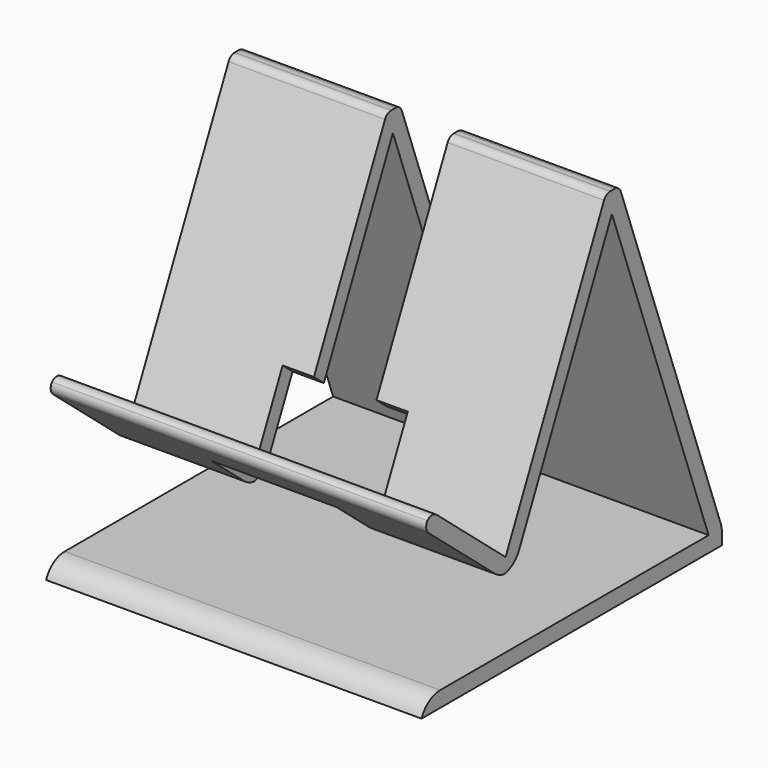
from build123d import *

# Parameters (mm, degrees)
F0_W        = 76.2
F0_H        = 76.2
F1_DEPTH    = 3.175
F3_DEPTH    = 76.2
F4_R        = 1.7145
F5_R        = 5.08
F6_T1_DEPTH = 84.7725
F7_T1_DEPTH = 92.3815846245
F7_T3_DEPTH = 85.4448439504
F8_T1_DEPTH = 99.7464301965
F9_W        = 12.7
F9_H        = 76.2
F10_REACH   = 149.9425757938
F11_W       = 25.4
F11_H       = 19.8840972021
F12_DEPTH   = 19.05
F14_DEPTH   = 0.5
F16_DEPTH   = 0.5


# Not quite as in the source:
# - a fillet or chamfer that OpenCascade refuses, or shapes differently, is made with other operations: its cross-section is extruded or revolved along the edge and cut away or added


with BuildPart() as f1:
    # F0 (on Top) → F1 (new body)
    with BuildSketch(Plane.XY):
        with Locations((-12.8260315396, -9.7117862726)):
            Rectangle(F0_W, F0_H)
    extrude(amount=F1_DEPTH)

    # F2 (on face) → F3 (join)
    with BuildSketch(Plane(origin=(-50.9260315396, 0, 0), x_dir=(0, -1, 0), z_dir=(-1, 0, 0))):
        Polygon((1.0524856216, 74.7795777039), (-0.4832286212, 70.560237499), (24.3855203494, 17.2290332271), (27.8887452421, 17.2290332271), (26.4995982243, 20.2080686204), align=None)
        Polygon((45.3054234366, 35.98802962), (26.4995982243, 20.2080686204), (27.8887452421, 17.2290332271), (47.3462740973, 33.5558385131), align=None)
        Polygon((-2.326278806, 74.7795777039), (-28.3882137274, 3.175), (-25.0094492998, 3.175), (-0.4832286212, 70.560237499), (1.0524856216, 74.7795777039), align=None)
    extrude(amount=-F3_DEPTH)

    # F4
    f4_edges = [f1.edges().sort_by_distance(p)[0] for p in [
        (-12.826032, -1.052486, 74.779578),
        (-12.826032, 2.326279, 74.779578),
    ]]
    fillet(f4_edges, radius=F4_R)

    # F5
    f5_edges = [f1.edges().sort_by_distance(p)[0] for p in [
        (-12.826032, 28.388214, 3.175),
    ]]
    fillet(f5_edges, radius=F5_R)

    # F6: fillet of radius 1.7145 on 2 edges, made by hand

    # F6_s2 → F6_t1 (cut)
    with BuildSketch(Plane.YZ.offset(-55.2122815396)):
        with BuildLine():
            ThreePointArc((-43.9920402389, 34.8859702632), (-45.2435281166, 35.2805628753), (-46.4074827934, 34.6746464223))
            Line((-46.4074827934, 34.6746464223), (-45.3054234366, 35.98802962))
            Line((-45.3054234366, 35.98802962), (-43.9920402389, 34.8859702632))
        make_face()
        with BuildLine():
            ThreePointArc((-46.2442147405, 34.8692217108), (-46.6388073527, 33.6177338331), (-46.0328908996, 32.4537791563))
            Line((-46.0328908996, 32.4537791563), (-47.3462740973, 33.5558385131))
            Line((-47.3462740973, 33.5558385131), (-46.2442147405, 34.8692217108))
        make_face()
    extrude(amount=F6_T1_DEPTH, mode=Mode.SUBTRACT)

    # F7: fillet of radius 5.08 on 2 edges, made by hand

    # F7_s2 → F7_t1 (cut)
    with BuildSketch(Plane.YZ.offset(-59.0168238518)):
        with BuildLine():
            ThreePointArc((-27.6218372743, 17.2290332271), (-24.8923552639, 18.0246046823), (-23.0177937162, 20.1621324574))
            Line((-23.0177937162, 20.1621324574), (-24.3855203494, 17.2290332271))
            Line((-24.3855203494, 17.2290332271), (-27.6218372743, 17.2290332271))
        make_face()
    extrude(amount=F7_T1_DEPTH, mode=Mode.SUBTRACT)

    # F7_s4 → F7_t3 (cut)
    with BuildSketch(Plane.YZ.offset(-55.5484535148)):
        with BuildLine():
            ThreePointArc((-29.3051375093, 18.417527456), (-27.7772387801, 17.5353947135), (-26.039776452, 17.2290332271))
            Line((-26.039776452, 17.2290332271), (-27.8887452421, 17.2290332271))
            Line((-27.8887452421, 17.2290332271), (-29.3051375093, 18.417527456))
        make_face()
    extrude(amount=F7_T3_DEPTH, mode=Mode.SUBTRACT)

    # F8: fillet of radius 5.08 on 1 edges, made by hand

    # F8_s2 → F8_t1 (cut)
    with BuildSketch(Plane.YZ.offset(-62.6992466379)):
        with BuildLine():
            ThreePointArc((-43.1025002333, 3.175), (-45.9423065647, 2.3071134838), (-47.8117862726, 0))
            Line((-47.8117862726, 0), (-47.8117862726, 3.175))
            Line((-47.8117862726, 3.175), (-43.1025002333, 3.175))
        make_face()
    extrude(amount=F8_T1_DEPTH, mode=Mode.SUBTRACT)

    f10_end = Plane(origin=(-12.8260315396, -35.2458192316, 27.5470194418), x_dir=(0, 0.7660444431, -0.6427876097), z_dir=(0, 0.6427876097, 0.7660444431))
    # F9 (on face) → F10 (cut, up to a plane its end follows)
    with BuildSketch(Plane(origin=(0, 26.0878488821, 9.4952004691), x_dir=(-1, 0, 0), z_dir=(0, 0.9396926208, 0.3420201433))):
        with Locations((12.8260315396, 44.4847803173)):
            Rectangle(F9_W, F9_H)
    f10_long = extrude(amount=-F10_REACH, mode=Mode.PRIVATE)
    add(split(f10_long, bisect_by=f10_end, keep=Keep.TOP, mode=Mode.PRIVATE), mode=Mode.SUBTRACT)

    # F11 (on face) → F12 (cut)
    with BuildSketch(Plane(origin=(0, -3.0393149772, -3.6221145432), x_dir=(1, 0, 0), z_dir=(0, -0.6427876097, -0.7660444431))):
        with Locations((-12.8260315396, 35.2600788025)):
            Rectangle(F11_W, F11_H)
    extrude(amount=-F12_DEPTH, mode=Mode.SUBTRACT)

    # F13 (on face) → F14 (cut)
    with BuildSketch(Plane(origin=(0, 26.0878488821, 9.4952004691), x_dir=(-1, 0, 0), z_dir=(0, 0.9396926208, 0.3420201433))):
        with BuildLine():
            add(Edge.make_bspline(
                [(-12.2205680236, 36.9647596645), (-12.4375809219, 37.1777145199), (-14.2561401515, 36.3922801097), (-16.3794366138, 36.048782003), (-17.5254932693, 36.3657786842), (-18.3014633617, 37.2696901613), (-17.2863519244, 37.2523004844), (-14.4576566032, 37.4954207878), (-11.5658920671, 37.805416436), (-10.6630117703, 37.9464776805), (-10.9800970944, 39.1793466969), (-10.7912415306, 41.042166104), (-11.8135815959, 41.4292498118), (-11.163322955, 42.1471276625), (-10.1032259508, 41.8804767346), (-8.5728479931, 41.3471502106), (-8.6405770888, 40.5582665139), (-9.0822908637, 39.9713628596), (-9.2936061196, 39.2829711537), (-9.3547227994, 38.2862647402), (-8.4949424153, 38.2939387249), (-6.2894265773, 38.7612641135), (-4.4550862415, 39.3336934473), (-3.5358588775, 39.4146215165), (-1.8897889247, 39.2197529843), (-1.0367428001, 38.634984577), (-0.9511188603, 37.964660191), (-1.7223036673, 37.4597752), (-3.473237626, 37.610469089), (-5.396188888, 37.4964088475), (-7.8020514484, 37.1779190401), (-9.2083980333, 37.4221742647), (-9.303619709, 36.5112671469), (-6.6590831045, 34.5799413955), (-4.7562674524, 32.7532527624), (-2.3354695053, 31.1292025084), (0.9361527089, 29.8634291742), (3.1927259884, 29.448658498), (4.7298825885, 29.1792840717), (5.1127190187, 28.7794124688), (4.6200426796, 28.242376998), (2.4432058563, 28.1653174305), (-2.0501291466, 27.8794533381), (-2.3021446512, 28.1846937913), (-3.4373326765, 29.0327348253), (-5.3275558013, 31.0433712554), (-7.7706651116, 33.5167964914), (-8.9965041632, 35.7672706229), (-9.3836795772, 35.832261965), (-9.5073061865, 35.2640611282), (-9.3215190458, 32.4732064417), (-9.3293575593, 28.7306751937), (-9.1248104107, 26.1783730415), (-9.5411467801, 25.1003176236), (-9.9939901766, 24.2566959019), (-10.3880489816, 24.159497297), (-10.6376358937, 24.4722289236), (-11.2202625154, 25.5509285761), (-11.6294601243, 26.6530189437), (-11.4594889103, 27.5804754259), (-11.0219047634, 28.6167282922), (-10.8093698167, 31.1236888801), (-10.6495633559, 33.8136680029), (-10.4829881905, 35.6308818012), (-10.8713651173, 35.7691549732), (-10.9488799824, 35.3596623296), (-13.0611611754, 32.0241729626), (-15.6128008079, 30.0939638419), (-17.8516788438, 28.6531090971), (-20.6329374247, 27.4418373755), (-21.6545938279, 27.2783643221), (-21.8006646214, 27.6856304921), (-21.2495727148, 27.9428385501), (-19.758792512, 28.571591964), (-17.1505064043, 30.6357950737), (-15.3240944139, 32.2157391856), (-13.3909983534, 34.5352022631), (-12.5076843563, 35.7085254148), (-12.0576365591, 36.8048749446), (-12.2205680236, 36.9647596645)],
                knots=[0, 0, 0, 0, 0.0149185043, 0.0314409106, 0.0431464978, 0.0527474566, 0.0608746499, 0.0796978372, 0.098409507, 0.1068890906, 0.1181168419, 0.1326566218, 0.1418086414, 0.150074082, 0.1614398511, 0.1745988579, 0.1829243593, 0.191996839, 0.201427718, 0.2110662413, 0.2195350999, 0.2360166609, 0.2509710776, 0.2613247706, 0.2750334233, 0.2856536419, 0.2933747425, 0.302723626, 0.3167744142, 0.3320931297, 0.34917677, 0.3608234741, 0.3683663313, 0.3873061139, 0.4054642032, 0.4236696503, 0.4437965392, 0.4604384593, 0.4734964468, 0.4801256596, 0.4873855353, 0.5039034485, 0.5264220872, 0.532589765, 0.5445465591, 0.5626750731, 0.5836043885, 0.6000683692, 0.6049107399, 0.6117052466, 0.6295128163, 0.6511594363, 0.6680475372, 0.6795050966, 0.6896706816, 0.6955735326, 0.7017785991, 0.7137294236, 0.7255074588, 0.7355193545, 0.7467040861, 0.763641916, 0.7822242342, 0.7958264928, 0.8006573208, 0.8061919669, 0.8270691209, 0.8470156738, 0.8647325217, 0.883551341, 0.8934192363, 0.8987085202, 0.9060579556, 0.9197511017, 0.9393419416, 0.9566280488, 0.9749391466, 0.988799312, 1, 1, 1, 1], degree=3))
        make_face()
        with BuildLine():
            add(Edge.make_bspline(
                [(-19.0648827702, 39.5692144203), (-19.202478136, 39.1142585113), (-19.5581018791, 38.5421318894), (-20.3428918902, 37.5263817898), (-21.2310155021, 37.1317217573), (-21.7154203892, 38.0693827698), (-21.9305391759, 38.899390242), (-21.7048788249, 39.9681885376), (-20.9430876784, 41.2228020945), (-20.0696984837, 42.191521594), (-19.8622909574, 43.2203731395), (-19.8676850202, 43.8805469393), (-19.3489828575, 43.9754783592), (-19.0078821058, 43.5626791427), (-18.7766646678, 42.8322849389), (-17.8190513756, 42.8642250168), (-14.894857764, 43.1656252037), (-11.9794175752, 43.6243620026), (-9.7917276455, 43.7435088922), (-7.2313882277, 44.0343683677), (-5.519610476, 44.2549316447), (-2.6518459565, 44.7628688356), (-1.1738872552, 45.0921410068), (-0.0100984334, 45.5409466088), (0.873304004, 45.2960716493), (1.6982131269, 44.7386312302), (2.8597230206, 44.0672740949), (3.6641541698, 43.2988812997), (4.0735853148, 42.7573362459), (3.8970171896, 42.132782947), (2.6234383732, 41.9394819935), (1.7878392935, 41.9359936575), (0.8885540736, 41.6152147558), (-0.1227543222, 41.1849641127), (-0.898150755, 40.6460777157), (-1.3031536017, 40.3461875672), (-1.7242571897, 40.8555116418), (-0.8211612167, 41.5326497088), (-0.214488068, 42.345648177), (-0.1218440174, 43.1060937664), (-0.6066845679, 43.8359563142), (-4.4627317829, 43.2283718237), (-6.8026668281, 43.1559679791), (-9.573337496, 42.8731130853), (-11.6444517647, 42.6894287813), (-14.7773676569, 42.4051995904), (-17.1993103247, 42.0974629023), (-18.4319703243, 42.0434725317), (-18.7473904838, 42.0491483936), (-18.714532473, 41.4716051199), (-18.8857390378, 40.1615490469), (-19.0648827702, 39.5692144203)],
                knots=[0, 0, 0, 0, 0.0200809179, 0.0408223728, 0.0568425282, 0.0740068898, 0.0912794902, 0.110126663, 0.1325366374, 0.153668939, 0.1724371044, 0.186345075, 0.1975998619, 0.2106719801, 0.2256738916, 0.2419864338, 0.273774106, 0.3060217213, 0.3335339044, 0.3625275885, 0.3874925255, 0.4186678058, 0.4418776195, 0.4617503709, 0.4787369469, 0.4971065061, 0.5186538966, 0.5382605755, 0.5527501686, 0.5655706602, 0.5857282106, 0.6030841453, 0.6207599759, 0.6403808777, 0.6584994033, 0.6702516694, 0.6817363332, 0.7000459733, 0.7191508485, 0.7343826384, 0.7488490189, 0.7840329922, 0.8141869545, 0.8440372542, 0.8710066867, 0.9037554013, 0.9333086705, 0.9530322314, 0.9613626963, 0.973855438, 1, 1, 1, 1], degree=3))
        make_face()
        with BuildLine():
            add(Edge.make_bspline(
                [(-14.6552044898, 47.7858823407), (-14.3287949418, 47.849008811), (-13.7342251747, 48.0187927188), (-13.1176794426, 47.7211387143), (-13.1258992772, 46.5583739408), (-13.0078974826, 45.7528080463), (-12.6705065264, 44.9246022715), (-12.3071563152, 44.6880030857), (-11.8375730204, 45.2237038894), (-11.8389448099, 46.1976678521), (-11.8208494214, 47.085636434), (-11.7717985904, 47.7375911908), (-11.8269555444, 48.2175236619), (-11.1382763912, 48.3098260396), (-9.8723263503, 48.485208953), (-8.3708221064, 48.6216779203), (-7.2601435678, 48.7700959102), (-7.0787470658, 48.4655937831), (-7.3793444834, 47.4247281921), (-7.7206266399, 46.3638172751), (-8.0832618313, 45.5629044956), (-8.0948415318, 45.0163155957), (-7.6095006048, 45.0268046247), (-6.9381896377, 45.729469285), (-6.3735174014, 46.6346442592), (-5.593587183, 47.9611719551), (-5.4450137868, 48.8743304375), (-4.7361482699, 49.0584433777), (-3.8262015976, 49.0540688613), (-2.2475496424, 49.0573366138), (-0.5905476412, 49.1110006163), (0.3761569662, 48.9895406059), (0.536197734, 49.3876679785), (0.6139251682, 50.0255318891), (-0.0567785878, 50.4030177805), (-0.7809724105, 50.8415422221), (-1.9942303434, 50.8260062138), (-2.7988194006, 50.7059482832), (-3.8263424891, 50.4935391094), (-4.4684864403, 50.1028246297), (-4.6680684813, 50.9185759427), (-4.0217427041, 51.8456088704), (-3.380821199, 52.8786532201), (-3.8037646999, 53.6018511109), (-4.5389467207, 53.9253035496), (-5.2135664575, 54.1037706185), (-6.0866887556, 54.5472224152), (-6.8435569559, 54.371907445), (-6.7978434329, 53.7317764983), (-6.5775575376, 53.3101437857), (-6.4906568549, 52.1489262847), (-6.4214330833, 50.8444945402), (-6.6037147523, 49.8522965378), (-7.8057430963, 49.6696898824), (-9.5197689724, 49.5022752972), (-10.8120866259, 49.4227011609), (-11.6404408204, 49.2821596419), (-11.963716563, 49.5578036849), (-11.9397081629, 50.5185117872), (-11.8410111727, 51.5657223735), (-12.1461390909, 51.8534408601), (-13.0795996704, 52.5546814101), (-13.9269942067, 52.797766627), (-15.1704479073, 52.9430477011), (-15.3025815763, 52.5032619508), (-15.3609842012, 52.2070750412), (-14.7638010704, 51.772011921), (-14.412957005, 51.3623994862), (-14.0538772902, 50.4985203483), (-13.6373676069, 49.329381939), (-14.0639260481, 48.8365960124), (-15.5768285452, 48.8596380194), (-17.2712284977, 48.7552146971), (-18.8981252056, 48.7552884082), (-19.3140274186, 48.5287421782), (-19.2539558575, 48.0415874229), (-18.6534702461, 47.6801503199), (-17.8289514003, 47.1102494485), (-17.1332173018, 47.1485649961), (-16.4106448716, 47.3528744088), (-15.5993894969, 47.6649880402), (-14.9839032929, 47.7223131364), (-14.6552044898, 47.7858823407)],
                knots=[0, 0, 0, 0, 0.0133526187, 0.0234217424, 0.0375677514, 0.0505814116, 0.0632896898, 0.0709832008, 0.0812702754, 0.0949294095, 0.1080654056, 0.1192361788, 0.1275957975, 0.1377851185, 0.1535643354, 0.1711329644, 0.184864659, 0.1914378111, 0.2053352153, 0.2204335045, 0.2333966027, 0.2422195377, 0.2500969199, 0.2632891978, 0.2779523312, 0.2950375212, 0.3075906437, 0.3182395875, 0.3313155675, 0.3487156615, 0.3669138188, 0.3794702083, 0.3874666809, 0.3977645807, 0.4091322754, 0.4219005583, 0.436685221, 0.4493783663, 0.4636032181, 0.4739082443, 0.4841052134, 0.4989987744, 0.5136936389, 0.5251445402, 0.5371881936, 0.5488374078, 0.5624143805, 0.5732091734, 0.5829776316, 0.5924911842, 0.6071166314, 0.6232621328, 0.6358400534, 0.6499936464, 0.6683773175, 0.6843460204, 0.6963212815, 0.7040474439, 0.7174585329, 0.7313263067, 0.7397880816, 0.7541715172, 0.7679524103, 0.7823537182, 0.7904046178, 0.797387364, 0.8086337485, 0.8188614885, 0.8323088317, 0.8472063495, 0.8566773008, 0.8729706061, 0.8918339881, 0.9090782731, 0.9173889209, 0.9257381783, 0.9371574856, 0.9508404908, 0.962005778, 0.9738077006, 0.9865537335, 1, 1, 1, 1], degree=3))
        make_face()
        with BuildLine():
            add(Edge.make_bspline(
                [(28.8704819977, 38.5385905075), (28.6669015037, 38.600319653), (28.3345652721, 38.884865852), (27.6662480137, 38.6701336841), (26.4686178944, 37.1758370499), (24.7462492926, 36.0245249499), (23.0241475487, 35.068401014), (22.0504692654, 34.8426951958), (21.3415008397, 34.3866820779), (20.9875014536, 34.7646305415), (21.7615759583, 35.1275787354), (23.1619603504, 36.1614495965), (24.9140251886, 37.4699567232), (26.5829353118, 39.2938967849), (27.8812000268, 40.7352801563), (29.0087562647, 42.6664898768), (29.3011369612, 43.5747853575), (29.6641666276, 44.3709519059), (29.3371185493, 44.4821206207), (27.7780683975, 44.1647561566), (25.9152727276, 43.5605143002), (25.2113587894, 43.6101263476), (23.7077362195, 44.2081835122), (23.4856932772, 44.5713497451), (23.7273941232, 45.1568891511), (26.0942814403, 45.1337781668), (28.8772270606, 45.2665339882), (30.8354311519, 45.7667843236), (33.6433327087, 45.8983428731), (34.6774169963, 46.0599402479), (35.6641990625, 46.0821283319), (36.3615362578, 46.7740142865), (37.0905947976, 47.7870189127), (38.0273561606, 49.1882469835), (38.4425149067, 50.5559077783), (38.7507748441, 51.5217016184), (38.5578841059, 52.3318516529), (38.8020639699, 52.3662048434), (39.4280391552, 52.4081584871), (40.3258899481, 51.7210417913), (40.8923263975, 51.036643167), (40.9856536964, 50.3423973884), (40.5304009498, 49.8043490605), (39.4187207, 49.0741307199), (38.3266564662, 47.9956583423), (37.8916464627, 47.4072677646), (37.0954683969, 46.7317136978), (37.1882183522, 46.2960444817), (38.5677518984, 46.4814344601), (40.0208453399, 46.9507033268), (41.9669973869, 47.1457090702), (43.1652732722, 47.1701756521), (43.8871701967, 46.5881994854), (44.5814988678, 45.9947460184), (44.5558114309, 45.629105085), (42.9722543673, 45.5976739248), (40.181089169, 45.6422990786), (36.8280213881, 45.4532441988), (36.5429548588, 45.3722110227), (36.6539550592, 44.9332282406), (38.791035876, 43.1757592482), (40.5618467279, 41.5482983991), (42.7754102606, 39.9523209145), (44.1177041414, 39.0492494347), (46.6979459927, 37.5558413082), (48.4083701574, 36.8534519629), (48.8096262688, 36.7241021633), (48.9086189009, 36.1350632824), (46.9443063883, 36.4486185947), (43.7453233674, 35.9038345104), (42.994365195, 36.8254972262), (40.9660108406, 38.5608908978), (40.3751599464, 39.6514549065), (39.8096422217, 39.8023086602), (38.6225812351, 39.5192094035), (37.1316287737, 39.2725491318), (34.4674186941, 39.035689323), (31.6606789821, 38.3468373354), (29.8545090997, 38.5809220218), (29.1219671578, 38.4623358344), (28.8704819977, 38.5385905075)],
                knots=[0, 0, 0, 0, 0.0088353791, 0.0174478263, 0.0329839413, 0.0499454579, 0.0657858899, 0.0773915649, 0.087176842, 0.0930738557, 0.1021923191, 0.1175005356, 0.13464786, 0.1524644191, 0.1687155693, 0.1854732029, 0.1971490329, 0.2067819655, 0.2117147744, 0.2261083078, 0.2422065381, 0.2521575768, 0.2663330571, 0.2731637712, 0.2804459354, 0.2973779594, 0.3168597403, 0.33347444, 0.35233753, 0.3641835998, 0.3749489244, 0.3858579619, 0.3986958363, 0.4135774702, 0.4272385695, 0.4389645262, 0.4484270969, 0.4528999034, 0.4615954444, 0.4737080717, 0.4845330496, 0.4934146081, 0.5024843686, 0.5158391246, 0.5299001908, 0.5401310004, 0.5513333399, 0.5569389353, 0.569369115, 0.5842378705, 0.6001772, 0.6123634924, 0.6233508221, 0.6339871866, 0.6390016865, 0.6518709335, 0.6726056949, 0.6930399068, 0.6977725647, 0.7038629509, 0.722417392, 0.7412345843, 0.759558213, 0.7743637177, 0.7942730527, 0.8096689683, 0.8164494264, 0.8225996572, 0.8375073043, 0.8580177211, 0.8700289446, 0.8886659849, 0.9011027809, 0.909009449, 0.9212390101, 0.9354255216, 0.9541730067, 0.9738148249, 0.9890855618, 1, 1, 1, 1], degree=3))
        make_face()
        with BuildLine():
            add(Edge.make_bspline(
                [(29.5810140669, 39.3035118151), (29.2471003406, 39.2833444534), (28.9096334838, 39.2817498274), (28.5302631206, 39.3155780135), (28.8665708276, 39.790595175), (29.5936321423, 40.7849440235), (30.266948503, 41.8352798964), (30.6801188854, 42.5794155683), (31.4736820946, 43.2865183591), (31.3751588249, 43.8377229052), (31.1125270077, 44.1714740085), (30.7777277841, 44.5291178142), (30.88549708, 44.8211300848), (31.3846159062, 44.9570804723), (32.5667034992, 44.933217921), (34.0192644877, 45.190064557), (35.5732949676, 45.3429369238), (35.9398414937, 44.7928555048), (37.2536186011, 43.8316707921), (38.1586780576, 42.4157505969), (39.447270883, 40.9526575395), (39.2906343528, 40.4754434928), (37.4657497136, 40.5402366875), (34.1861686574, 39.8820931682), (32.1335485609, 39.536224822), (30.1870464435, 39.340114306), (29.5810140669, 39.3035118151)],
                knots=[0, 0, 0, 0, 0.0352834971, 0.0547099565, 0.0808820836, 0.1280629153, 0.174256765, 0.2129085747, 0.2537479057, 0.2819512633, 0.3091699939, 0.3368908858, 0.3565079542, 0.3842326188, 0.4286781072, 0.4808663893, 0.5297961617, 0.5610670087, 0.6118310381, 0.6685943478, 0.7239360366, 0.7451249293, 0.7974249871, 0.8739701091, 0.9359626757, 1, 1, 1, 1], degree=3))
        make_face(mode=Mode.SUBTRACT)
        with BuildLine():
            add(Edge.make_bspline(
                [(32.5110442936, 27.8633278477), (32.0797348479, 27.8533306779), (31.5480401004, 27.8520912257), (30.9840187704, 27.6425406267), (30.8204208637, 26.8192396271), (30.6283837261, 26.4391585676), (29.8864102772, 26.5818420698), (29.7062382905, 28.2653008664), (29.3365553938, 30.259336559), (28.7292119902, 31.2527871479), (28.4335540173, 31.5239320875), (28.4396648665, 32.507671209), (29.3799558832, 32.2709307134), (30.4020991802, 31.7653251756), (31.2540623001, 31.4058174865), (32.8338495564, 31.7323439823), (34.6820855203, 32.17044277), (36.3538851241, 32.6484665595), (37.1309726039, 32.887865034), (38.4772796994, 32.6555121008), (39.5119414906, 31.8078800594), (40.0624138682, 31.4669663606), (39.6327249342, 30.6423379425), (38.8275529363, 29.9222079693), (38.3776732467, 29.6032263974), (38.4052502513, 29.0390934053), (38.7614544378, 29.003379106), (38.7141421192, 28.1079722967), (37.4515054144, 28.1504564858), (35.226260608, 27.9601637407), (33.2188514413, 27.8797338605), (32.5110442936, 27.8633278477)],
                knots=[0, 0, 0, 0, 0.0347896695, 0.0595448855, 0.0905872612, 0.1116397569, 0.1361291141, 0.1797743453, 0.2312124895, 0.2671577228, 0.2891404641, 0.3184718202, 0.3481097286, 0.3861910907, 0.418954181, 0.4620634472, 0.5115463244, 0.5568298434, 0.5878724886, 0.6276388622, 0.6682882335, 0.6930167736, 0.7236806106, 0.7607217447, 0.7860726928, 0.8089504055, 0.8267380365, 0.8537265595, 0.8890282467, 0.9429078659, 1, 1, 1, 1], degree=3))
        make_face()
        with BuildLine():
            add(Edge.make_bspline(
                [(33.7959080935, 31.204862954), (34.3256433285, 31.2598558637), (34.9989774326, 31.389734461), (36.1267733135, 31.6375209475), (36.6540315864, 31.342401281), (36.8108571179, 30.4821973307), (36.7830604953, 29.5522133198), (36.1142583817, 29.1006750432), (34.2934736329, 28.9977869009), (32.3635644811, 28.755375729), (31.5827800422, 28.5972541539), (30.8369526476, 28.5711827688), (30.7907732292, 29.5276281022), (30.5547142961, 30.7691675903), (31.4530298238, 31.0521102912), (33.0764838908, 31.1301780406), (33.7959080935, 31.204862954)],
                knots=[0, 0, 0, 0, 0.0794716815, 0.1511738761, 0.2004647424, 0.2642103714, 0.3293682538, 0.3863654984, 0.4809996427, 0.5793228837, 0.6420814562, 0.6937732674, 0.7578967126, 0.8321030051, 0.8920708926, 1, 1, 1, 1], degree=3))
        make_face(mode=Mode.SUBTRACT)
        with BuildLine():
            add(Edge.make_bspline(
                [(34.2563502491, 33.6589482296), (33.7282921419, 33.5983778563), (31.8223582272, 33.5935145232), (30.9038275344, 33.5665464268), (30.4145775555, 33.7649939084), (30.5447020395, 34.4281162513), (32.474261405, 34.5234464535), (34.466015289, 34.9599666727), (36.1791114632, 35.0849534737), (37.3651732942, 35.2545267586), (37.5817088924, 34.5600136201), (37.0064808731, 34.2986205856), (34.822425888, 33.8258988568), (34.5364561971, 33.6910775002), (34.2563502491, 33.6589482296)],
                knots=[0, 0, 0, 0, 0.1224650275, 0.2013629669, 0.2507008551, 0.3008222594, 0.4053293725, 0.5223282297, 0.627352239, 0.7075993931, 0.7608387042, 0.8188217478, 0.9350390001, 1, 1, 1, 1], degree=3))
        make_face()
        with BuildLine():
            add(Edge.make_bspline(
                [(32.0696309209, 36.1306820679), (32.8290956828, 36.1058081386), (34.3707662839, 36.1197979256), (36.8293427492, 36.6963124833), (37.5250700117, 37.1013598316), (37.4095991975, 37.6008901688), (36.9921531792, 37.983267452), (35.0356242187, 37.6047169294), (33.3618681033, 37.2036261493), (31.9974126364, 36.9578288162), (30.8530613817, 37.1876503098), (30.2025637815, 36.746803603), (30.5337327041, 36.2122161684), (31.4560095571, 36.1507793458), (32.0696309209, 36.1306820679)],
                knots=[0, 0, 0, 0, 0.1199751121, 0.2432717129, 0.306190792, 0.3548365531, 0.4075425814, 0.5144736702, 0.6203673051, 0.7112286011, 0.7945893349, 0.854173685, 0.9030642426, 1, 1, 1, 1], degree=3))
        make_face()
        with BuildLine():
            add(Edge.make_bspline(
                [(28.8852266967, 47.9994755852), (29.0365112874, 47.8170923521), (29.471421325, 47.3088430928), (30.03935622, 46.9041701683), (30.6573571332, 47.1228232889), (30.8313945201, 48.4906663343), (30.2759854906, 49.4598405131), (29.2005293678, 49.8662684429), (28.4785969703, 50.5110796541), (27.8638906667, 50.2309325537), (28.1401522934, 49.4498183455), (28.605600629, 48.347971072), (28.778277948, 48.1284091301), (28.8852266967, 47.9994755852)],
                knots=[0, 0, 0, 0, 0.0958238879, 0.1779780076, 0.2483251988, 0.3608211602, 0.4648763121, 0.5725271629, 0.6686051265, 0.7351776133, 0.8215018734, 0.9322585013, 1, 1, 1, 1], degree=3))
        make_face()
        with BuildLine():
            add(Edge.make_bspline(
                [(32.9267159104, 49.395174222), (33.1108905307, 49.0481035082), (33.3649874075, 48.4629871598), (34.2495684033, 47.8435255745), (34.9575467185, 48.1828327096), (35.3143062262, 48.8704691554), (35.2217551683, 49.7996485449), (34.3862566398, 50.4974324905), (33.5047664739, 50.9107158801), (32.5164681408, 51.2502770484), (32.1009003705, 51.0117603368), (32.2915343846, 50.4844457673), (32.7219494476, 49.7810495522), (32.9267159104, 49.395174222)],
                knots=[0, 0, 0, 0, 0.1027534347, 0.1993841047, 0.2807279369, 0.3659768547, 0.4582794021, 0.5590952596, 0.6608207011, 0.7607221056, 0.8182593378, 0.8857581065, 1, 1, 1, 1], degree=3))
        make_face()
    extrude(amount=-F14_DEPTH, mode=Mode.SUBTRACT)

    # F15 (on face) → F16 (join)
    with BuildSketch(Plane(origin=(0, 26.0878488821, 9.4952004691), x_dir=(-1, 0, 0), z_dir=(0, 0.9396926208, 0.3420201433))):
        with BuildLine():
            add(Edge.make_bspline(
                [(-18.067419529, 11.0000511631), (-18.0294524157, 10.7235310227), (-17.875867252, 10.0109918698), (-19.2710762763, 10.1793831628), (-20.593468805, 9.7637410417), (-21.019457124, 10.0355451772), (-21.5089096437, 10.1228416118), (-21.9608158739, 10.1029552012), (-22.0577140792, 9.8667785234), (-21.588670436, 9.3757485124), (-21.1388639716, 8.4792945583), (-20.9236895852, 7.4896480722), (-20.6834398601, 6.79169381), (-20.5022720201, 6.2579548773), (-20.2901775921, 6.1015687253), (-20.098101844, 6.2663451169), (-20.0987359315, 6.5704923134), (-19.850442274, 6.8106368009), (-19.1439382254, 6.7335576195), (-18.6649835595, 6.922685976), (-18.2679950739, 6.9939030432), (-17.9785858791, 7.0808172904), (-18.041290729, 6.3268239176), (-18.0565132814, 5.5770954783), (-17.9449866152, 5.2434714022), (-17.7998107047, 5.1092310439), (-17.4880528726, 5.6859626382), (-17.303658295, 6.3747558873), (-17.200042047, 6.859787816), (-17.2628283372, 7.1641612454), (-16.7464645603, 7.1715460723), (-16.0037134146, 7.2488787731), (-15.3454264031, 7.2722523327), (-14.6339931171, 7.3668145206), (-14.4210832539, 7.5302895663), (-14.5146307339, 7.8624759362), (-14.7774182016, 7.9461970506), (-14.4556120371, 8.4023349662), (-13.8827892489, 9.0167292162), (-13.376494058, 9.5090916559), (-13.0983115784, 9.855457924), (-13.1295141866, 10.131986632), (-13.9239636397, 10.620706995), (-14.6373731205, 11.0492042252), (-15.2746498895, 11.1222787389), (-16.4622150344, 10.629787861), (-16.9905237743, 10.4466394942), (-17.231677203, 10.4348044471), (-17.1680261714, 11.0555372639), (-17.1819576986, 11.8206809892), (-16.8959183664, 12.5161789364), (-17.0193238274, 12.9631968294), (-17.4694751822, 13.275443282), (-18.1539543084, 13.4193782185), (-18.4363271362, 13.3950070483), (-18.5318515351, 13.1262236708), (-18.3483851236, 12.7828855661), (-18.1192672916, 11.8010692298), (-18.1075374492, 11.2922359515), (-18.067419529, 11.0000511631)],
                knots=[0, 0, 0, 0, 0.0210238222, 0.0468944869, 0.0756072012, 0.0918333629, 0.1090031803, 0.1246288474, 0.1343744807, 0.1533376265, 0.1781711863, 0.2026421249, 0.22376356, 0.2416933917, 0.2525670218, 0.2632656071, 0.2762686929, 0.2893309417, 0.3093335709, 0.3271042833, 0.3425847172, 0.3529702674, 0.372154051, 0.394276255, 0.408138488, 0.416022284, 0.4338940152, 0.4555424342, 0.4725520036, 0.4838400478, 0.4993982468, 0.5208348891, 0.5411896738, 0.5614074045, 0.572695613, 0.5857546976, 0.5963227543, 0.6122159327, 0.6353340346, 0.6560851869, 0.6714618604, 0.6825436579, 0.7054962419, 0.7279418344, 0.7469530775, 0.7745037773, 0.7927558508, 0.8018647712, 0.8192998601, 0.8415309681, 0.8621464713, 0.8775644948, 0.8952286706, 0.9155972317, 0.9275873259, 0.9388503623, 0.9537223413, 0.9777851949, 1, 1, 1, 1], degree=3))
        make_face()
        with BuildLine():
            add(Edge.make_bspline(
                [(-20.4448979348, 8.5930200294), (-20.4920795431, 8.703217197), (-20.608796905, 8.994646863), (-20.685605748, 9.5354052653), (-19.8620466081, 9.4725768265), (-19.0731185629, 9.6823382068), (-18.0097317579, 9.9092100947), (-18.1119347333, 9.2915345388), (-18.0884238445, 7.5312970203), (-18.046113917, 7.3624679064), (-18.8051761657, 7.3359636489), (-19.5340356917, 7.1792311755), (-20.0034564872, 7.0777846795), (-20.105886291, 7.4045992451), (-20.3223634914, 8.3251180874), (-20.4058401507, 8.5017968316), (-20.4448979348, 8.5930200294)],
                knots=[0, 0, 0, 0, 0.062049316, 0.1206961092, 0.1950159752, 0.2860209161, 0.3716640642, 0.4357861542, 0.5601565875, 0.5905623197, 0.665713993, 0.7515382806, 0.8089187876, 0.8583517115, 0.94863446, 1, 1, 1, 1], degree=3))
        make_face(mode=Mode.SUBTRACT)
        with BuildLine():
            add(Edge.make_bspline(
                [(-17.1649176627, 8.1401150674), (-17.1717711853, 7.9904290571), (-17.1872617983, 7.7185017206), (-17.0166036283, 7.640894644), (-16.4428709258, 7.7459086533), (-15.8101724493, 7.9037039564), (-15.4256700112, 8.0137108346), (-15.2154402496, 8.6778649672), (-15.0652079927, 9.2342312273), (-15.0204570315, 10.019651498), (-15.1619378463, 10.3511576463), (-15.7497761877, 10.3102218815), (-16.3714581953, 10.1769865456), (-17.2005793262, 10.1068642523), (-17.1558347813, 9.8758226353), (-17.1472050494, 8.6737934031), (-17.1567093524, 8.3193906455), (-17.1649176627, 8.1401150674)],
                knots=[0, 0, 0, 0, 0.0585781604, 0.0921762, 0.1618308782, 0.2381318896, 0.2933275251, 0.3663394563, 0.4399564842, 0.5206578305, 0.5700526346, 0.6352477438, 0.7147912857, 0.7928054139, 0.8298206478, 0.9298422507, 1, 1, 1, 1], degree=3))
        make_face(mode=Mode.SUBTRACT)
        with BuildLine():
            add(Edge.make_bspline(
                [(-22.6708725095, 4.3283575214), (-22.7814406689, 4.0971394514), (-22.9963748342, 3.5436742203), (-23.5471646724, 2.6528075409), (-23.5447825072, 2.3472119366), (-23.6329464789, 1.6207698224), (-23.3810285543, 1.3664994771), (-22.8402240279, 1.6873896732), (-22.3705955908, 2.2793785009), (-22.0912474778, 2.9467235157), (-21.9593088376, 4.0257028457), (-22.1167379331, 4.8397226751), (-22.1944136871, 5.1174749569), (-22.4988030423, 5.0972689071), (-22.4350841693, 4.7709105507), (-22.5860377058, 4.5057624785), (-22.6708725095, 4.3283575214)],
                knots=[0, 0, 0, 0, 0.0899781937, 0.1857195513, 0.2410292704, 0.3207674475, 0.3689627503, 0.4396562246, 0.5237669746, 0.6052105823, 0.706010249, 0.7935168654, 0.839999411, 0.8824086997, 0.9309631052, 1, 1, 1, 1], degree=3))
        make_face()
        with BuildLine():
            add(Edge.make_bspline(
                [(-20.8503101021, 4.1725048795), (-20.8863381603, 4.3585987365), (-20.9083610316, 4.6004237723), (-20.8273431771, 4.8496471022), (-20.6230108503, 4.7470227087), (-20.2551440261, 4.3346003872), (-20.1652059536, 3.935824011), (-19.8592467362, 2.9006460177), (-19.0657664667, 1.8741877335), (-18.101397795, 1.2406055176), (-16.7783341889, 1.1100450329), (-15.4340431548, 1.0501217861), (-14.417730159, 1.3489172239), (-13.9967056517, 1.4761077672), (-14.0129822173, 1.7573873485), (-14.3921376732, 2.4947967059), (-14.7447034521, 2.9527779412), (-14.7139213058, 3.2478387575), (-14.5343557167, 3.3365214223), (-14.1850417836, 2.9490912244), (-13.5388155651, 2.3032535617), (-12.6499258944, 1.7838156892), (-12.0945276886, 1.6151093978), (-11.8657227146, 1.4802392806), (-11.7057720383, 1.1230736326), (-12.7959877627, 0.6595434107), (-14.259370023, 0.2502810741), (-15.9737254724, 0.3057875519), (-17.8761421334, 0.2775741658), (-18.708337893, 0.8019037353), (-19.4345339954, 1.231098086), (-20.2284239637, 2.2059610046), (-20.5895891619, 3.1716819702), (-20.7972836456, 3.8986100793), (-20.8503101021, 4.1725048795)],
                knots=[0, 0, 0, 0, 0.0247228787, 0.0404227264, 0.0552343594, 0.0818867134, 0.1054186641, 0.1425361279, 0.1842505885, 0.2226714689, 0.2642551678, 0.307167422, 0.344674877, 0.3664591447, 0.383163866, 0.4166203951, 0.4448049256, 0.4625648576, 0.4756834139, 0.5001060374, 0.5359530056, 0.5732934194, 0.6005749286, 0.6187897614, 0.6368162328, 0.6732158279, 0.7193103325, 0.7677162354, 0.8174244128, 0.8525069195, 0.8856216092, 0.9258299311, 0.9636126199, 1, 1, 1, 1], degree=3))
        make_face()
        with BuildLine():
            add(Edge.make_bspline(
                [(-17.9717317224, 4.1637541726), (-18.0877748202, 4.2841360964), (-18.3756074579, 4.5618798625), (-18.4375688841, 4.9545384824), (-18.1273350117, 5.0418397614), (-17.4747515979, 4.8245453583), (-16.7263653937, 4.3884884704), (-16.2910393605, 3.8857760347), (-16.193427401, 3.4162691235), (-16.6808811757, 3.0543392076), (-17.1802260034, 3.3891163839), (-17.7302202275, 3.8946880624), (-17.8790073902, 4.0675628981), (-17.9717317224, 4.1637541726)],
                knots=[0, 0, 0, 0, 0.0957731066, 0.1669003282, 0.2276697716, 0.331836836, 0.4516485728, 0.5535810709, 0.6342640922, 0.7203124569, 0.8144306044, 0.923472421, 1, 1, 1, 1], degree=3))
        make_face()
        with BuildLine():
            add(Edge.make_bspline(
                [(-13.6463306844, 5.2313683555), (-13.8325670083, 5.3868329253), (-14.1618541027, 5.6702263579), (-14.3720330292, 5.7700652436), (-14.3337234384, 6.0659018629), (-13.6056706378, 5.9624748166), (-12.5680533591, 5.8169077477), (-11.8870765524, 5.5970144586), (-11.3060671069, 5.0253390467), (-11.2053491988, 4.6545097387), (-11.1827522224, 4.0906101768), (-11.2972601399, 3.8549441215), (-11.8101531844, 3.8990453936), (-12.4235379861, 4.2671079436), (-13.1260938579, 4.8086189121), (-13.4624095673, 5.0778364516), (-13.6463306844, 5.2313683555)],
                knots=[0, 0, 0, 0, 0.0803505893, 0.1238353948, 0.1636772746, 0.2403324094, 0.3418295742, 0.4243127849, 0.5078001008, 0.5685575954, 0.639637447, 0.6836553871, 0.7470597082, 0.8302091736, 0.9206482933, 1, 1, 1, 1], degree=3))
        make_face()
        with BuildLine():
            add(Edge.make_bspline(
                [(-6.53333636, 5.3354469128), (-6.5386419385, 5.7015184529), (-6.5430803783, 6.5651211292), (-6.5343389774, 6.8297628366), (-6.7565729716, 6.8002443543), (-7.1719963812, 6.5283675016), (-7.9108208296, 6.0837757618), (-8.1597111031, 5.9795323795), (-8.7078124308, 5.9594008437), (-9.1861306407, 6.1885347791), (-9.3648212558, 6.3821268866), (-9.3209269091, 6.6741705811), (-8.9591072954, 6.7970021523), (-8.414948243, 6.7247797097), (-7.8005595314, 6.9535702451), (-7.0734230666, 7.2210477743), (-6.5382525682, 7.7717690374), (-6.3842347739, 8.0419852642), (-5.7952133748, 8.0360233385), (-5.3723607406, 7.8735882815), (-5.0626131526, 7.7128726194), (-4.8828037954, 7.5241268146), (-5.0304358356, 7.2478254225), (-5.5018081974, 6.9461265995), (-5.6572273748, 6.3226481515), (-5.9101920962, 5.4429388286), (-5.9667351348, 3.3113216118), (-5.9751084753, 3.0457500399), (-5.8921871949, 2.9477749962), (-5.7304115092, 3.2210317578), (-5.1558094975, 3.8272155907), (-4.6606181219, 4.2979999673), (-4.444221484, 4.4931761363), (-4.2504487376, 4.5932375029), (-4.213916775, 4.3971010054), (-4.3254246211, 3.9917022224), (-5.290757659, 2.8459212135), (-5.8819794813, 2.0903587489), (-6.613197352, 0.8431510189), (-6.7796597929, 0.6452667038), (-7.0759679887, 0.7080321456), (-7.3496348038, 1.210936441), (-7.4503269702, 1.457277949), (-7.5100522155, 1.8762582977), (-7.2034566203, 2.1372622424), (-6.7361030322, 2.6657593392), (-6.5634691686, 3.2748679084), (-6.5175724967, 4.747402889), (-6.5295638391, 5.0751524792), (-6.53333636, 5.3354469128)],
                knots=[0, 0, 0, 0, 0.0337856829, 0.0471450483, 0.0586250584, 0.0803700855, 0.1081840117, 0.1239672811, 0.1456199318, 0.1674905661, 0.1821166484, 0.1966077657, 0.213972588, 0.2360649513, 0.2601958415, 0.2870086334, 0.3127700476, 0.3286300031, 0.3504455345, 0.3711858051, 0.3888313937, 0.4026976407, 0.4179189439, 0.4399645734, 0.4627760188, 0.4930436858, 0.536632058, 0.5512630873, 0.5588712442, 0.5734510562, 0.6017498383, 0.6268685037, 0.6431556238, 0.6549972287, 0.6656367414, 0.6846133563, 0.720616802, 0.7526411786, 0.7877852895, 0.8017183224, 0.8163543365, 0.8386049631, 0.8548755415, 0.8729480476, 0.8914778247, 0.9159848907, 0.9405649748, 0.975976758, 1, 1, 1, 1], degree=3))
        make_face()
        with BuildLine():
            add(Edge.make_bspline(
                [(-3.0697847251, 3.8180698175), (-3.1741201778, 3.3509244175), (-3.476262536, 2.3018682929), (-4.4412200695, 1.1449139854), (-5.1364254039, 0.5708657907), (-5.4223052701, 0.5970308616), (-5.3384975964, 0.7851846934), (-4.9268383841, 1.2438723731), (-4.4530201348, 1.9378517998), (-4.0434867453, 2.8528651725), (-3.7382800258, 3.9817475488), (-3.4755166618, 5.0639357885), (-3.3661922255, 6.4879825873), (-3.5999455227, 7.2628169477), (-3.974644791, 7.897868246), (-3.937137577, 8.2454895848), (-3.7021920502, 8.4344565776), (-3.2758069924, 8.2390697532), (-2.7387809877, 8.0237837435), (-2.34300075, 8.1637951228), (-1.0932539558, 8.3265307803), (-0.6756485399, 8.5214903991), (-0.5864200791, 8.6367913656), (-0.9357036158, 9.5556472963), (-1.2313771922, 10.8263222007), (-1.2821041517, 12.0205605411), (-1.5442894586, 12.3185505167), (-1.9097477864, 12.6554314219), (-2.0418880563, 12.9059993729), (-1.9455399593, 13.2549987791), (-1.5656024595, 13.2291237188), (-1.0955136436, 13.2155160756), (-0.8299618705, 13.0317034609), (-0.2703826066, 12.8067208681), (-0.3256617929, 12.5228795307), (-0.4028549591, 11.1728653973), (-0.2878857642, 10.1890450168), (-0.0779811179, 8.7818705303), (0.0831768098, 8.6932556891), (0.612443029, 8.8173603519), (1.2519017414, 9.0889378359), (1.8507213418, 9.1374284649), (2.3640718824, 9.1244154832), (2.5870233648, 8.9632408462), (2.7205433164, 8.7961871852), (2.4953005077, 8.5915833834), (1.9399838887, 8.4089368463), (1.0810204578, 8.075562039), (0.2459287772, 8.1320624907), (0.2028100914, 7.9835336583), (0.458751144, 6.796568828), (0.8600839341, 5.4397482251), (1.1133352774, 4.4968677382), (1.2539176636, 4.2186141884), (1.4553968394, 4.1956492746), (1.4748308442, 4.6487227171), (1.8998244509, 5.4915051368), (1.9799838757, 6.8101191372), (1.7756352234, 7.3432586525), (2.2688323973, 7.3803636959), (2.7665932515, 7.2220393451), (3.1665328227, 6.7829093811), (3.1782368251, 6.6020985588), (3.1146522464, 6.2148449975), (2.7856955894, 5.876981323), (2.5117076118, 5.194267228), (2.1527216773, 4.3309151526), (1.6629673701, 3.6654321641), (1.6331598962, 3.4146716044), (2.597143187, 1.8919693273), (3.3150637186, 1.3056610264), (3.7149138146, 1.1114690154), (3.8770264501, 1.0517322071), (4.0519087062, 1.4235935403), (4.5940713466, 2.1733532234), (4.8110770895, 2.6985117488), (5.0121876494, 2.6864280224), (4.950538128, 2.0531654115), (4.8117999059, 1.168977112), (4.8972487902, 0.2595760969), (5.0657211889, -0.0915478713), (4.8243099725, -0.4178904439), (4.1553767114, -0.2616304161), (3.1987631447, 0.439048508), (2.1131607728, 1.420407813), (1.4620580807, 2.4084130554), (1.27534775, 2.7723987025), (1.2406151838, 2.9187521727), (1.009761548, 2.8045822342), (0.5317595492, 2.2052648958), (-0.2714625689, 1.597135539), (-1.2314520512, 1.2240343112), (-1.4999158668, 1.0766785665), (-1.6837203508, 1.1939369069), (-1.3703973538, 1.3237012322), (-0.7105827056, 1.850710502), (0.3049422581, 2.7709902132), (0.6977959198, 3.3119581216), (0.8968726601, 3.5852324697), (0.6855369489, 3.997851484), (0.2036902419, 5.3081964112), (-0.08964863, 6.3033699457), (-0.4534697984, 7.5667500601), (-0.4660825544, 7.8906865447), (-0.703484443, 7.9085002418), (-1.4811216119, 7.6863801623), (-2.5101226645, 7.5461861089), (-2.7864911889, 7.4157400476), (-2.698744011, 6.2912159547), (-2.7816321877, 5.8938504397), (-2.6904598065, 5.7650855573), (-2.3533225735, 5.7428245711), (-1.8313264031, 6.1523091238), (-1.3321548858, 6.3035608883), (-0.9063303332, 6.0843454148), (-0.4047223702, 5.7268733399), (-0.654170028, 5.3270697189), (-0.8290001149, 4.9509524085), (-0.7557529393, 4.0144434462), (-0.8832702024, 3.1782591108), (-1.3217154802, 2.2579220339), (-1.8340663434, 1.9557199324), (-2.0651584548, 2.0009143526), (-2.2097565451, 2.2821204127), (-2.407765121, 2.8452407535), (-2.6447445499, 3.1288558669), (-2.8180659119, 3.2316103241), (-2.7402230137, 3.4572192094), (-2.2983392876, 3.3303191814), (-2.1638382617, 3.2237062592), (-1.7120700569, 3.1859295474), (-1.532184491, 4.2476028319), (-1.4885742437, 5.1819710309), (-1.6202432145, 5.4244355601), (-1.960659987, 5.4283807785), (-2.6833937813, 5.1679488096), (-2.8907843931, 5.2000367366), (-2.9000442064, 4.7345745074), (-2.9859311453, 4.1935108879), (-3.0697847251, 3.8180698175)],
                knots=[0, 0, 0, 0, 0.0121062102, 0.0242383967, 0.0332327888, 0.0372904254, 0.0407977088, 0.0483926999, 0.0574405042, 0.06718425, 0.0776293144, 0.0880847988, 0.0995726877, 0.1084261132, 0.1165835279, 0.121976188, 0.1266728109, 0.1331687867, 0.1403904327, 0.1467627396, 0.1577696877, 0.1641625022, 0.1671328575, 0.1762180548, 0.1880310231, 0.1983453007, 0.2043103814, 0.2110432827, 0.2161731549, 0.2213146435, 0.2269699519, 0.2335704187, 0.2393229221, 0.2463862454, 0.2510807084, 0.2620385732, 0.2727877516, 0.2838462864, 0.2872967009, 0.2941761601, 0.302493654, 0.3100975746, 0.3169386792, 0.3219524967, 0.3258791746, 0.3305559567, 0.33799018, 0.3477633495, 0.356139346, 0.3589585562, 0.369273277, 0.3815665279, 0.3910345075, 0.396064764, 0.3994089992, 0.4051868488, 0.4148995623, 0.4262167505, 0.4325288503, 0.4382792492, 0.4455850368, 0.4527874426, 0.4568112654, 0.462618466, 0.4692331376, 0.4774992309, 0.4872381571, 0.4957523902, 0.5002947293, 0.5130980042, 0.5229452484, 0.5290674455, 0.5324245215, 0.5381045333, 0.5478934395, 0.5549287632, 0.5578582749, 0.5649408009, 0.5746653225, 0.5838891031, 0.5896484797, 0.5949019375, 0.6023707006, 0.6130453532, 0.625088693, 0.6356460045, 0.6416532097, 0.6446837308, 0.648775078, 0.6572349284, 0.6673558547, 0.6771844615, 0.6823203192, 0.685635457, 0.6901757485, 0.6993449637, 0.7109490892, 0.7188743013, 0.7239329517, 0.7301338975, 0.7415180761, 0.7521110414, 0.7631139291, 0.7680178761, 0.7719258976, 0.7808607909, 0.7908355041, 0.7955642401, 0.8056761104, 0.8119149592, 0.8151559719, 0.8203614489, 0.8283193863, 0.8351428096, 0.8418568196, 0.8488971783, 0.8548133023, 0.8611021086, 0.8703274514, 0.8795218933, 0.8892683712, 0.8964087826, 0.9005709797, 0.9058328118, 0.9134656676, 0.9193993862, 0.9233855116, 0.9271040926, 0.9332532177, 0.9375687159, 0.9429197673, 0.952628114, 0.9622383421, 0.9666285043, 0.9720695005, 0.9806712415, 0.9844589483, 0.9902703344, 1, 1, 1, 1], degree=3))
        make_face()
        with BuildLine():
            add(Edge.make_bspline(
                [(1.0175870266, 10.9123811126), (0.9248001212, 10.971406486), (0.7605424553, 11.0310114577), (0.7788429911, 11.3288643458), (1.2264820604, 11.3356262757), (2.0950812161, 11.3298725669), (2.5874083078, 11.0253294995), (2.9333944752, 10.7745509914), (2.9182307119, 10.3301218684), (2.8824192346, 10.0159022295), (2.4393663386, 10.0039877438), (2.0270656103, 10.1901816918), (1.4456572191, 10.5336164477), (1.1510634328, 10.827471559), (1.0175870266, 10.9123811126)],
                knots=[0, 0, 0, 0, 0.0658248279, 0.1207254893, 0.1987463951, 0.3179529762, 0.4139849695, 0.4923693524, 0.5740859452, 0.6389060193, 0.7143912034, 0.8009653856, 0.905309252, 1, 1, 1, 1], degree=3))
        make_face()
        with BuildLine():
            add(Edge.make_bspline(
                [(-6.3614849932, 10.5106672272), (-6.5059183708, 10.6154879494), (-6.9945328189, 11.0369235942), (-7.0259729582, 11.2691833542), (-6.749090783, 11.3997680662), (-5.7659393995, 11.3606403541), (-5.1556181644, 11.0004209693), (-4.6538318324, 10.6511760011), (-4.6703386983, 10.1317606453), (-4.8634683883, 9.8067768765), (-5.2218889254, 9.7740814043), (-5.6863703495, 9.9467000637), (-6.2162648939, 10.4347868597), (-6.2934551599, 10.4612954242), (-6.3614849932, 10.5106672272)],
                knots=[0, 0, 0, 0, 0.1102381592, 0.1621308741, 0.221781711, 0.3415347405, 0.4471167114, 0.5378987312, 0.6210817569, 0.6922588267, 0.7599605877, 0.8479969999, 0.94807652, 1, 1, 1, 1], degree=3))
        make_face()
        with BuildLine():
            add(Edge.make_bspline(
                [(22.1921242774, 2.1906606853), (21.8399618059, 2.1244288186), (21.24476373, 2.012488783), (20.767103753, 2.0823114613), (20.2080949831, 2.4615966988), (19.8308166094, 2.7507412294), (19.7783639858, 2.8743256974), (20.2162283962, 2.8757123135), (21.6588672863, 2.8723786617), (23.2251465538, 3.030977461), (24.1937953158, 3.1646622989), (24.4470417936, 3.2357413182), (24.4448236066, 3.3612382408), (24.4192549033, 4.8108119435), (24.4364060258, 6.1826563599), (24.4165129856, 7.7417235886), (24.3827248921, 8.4279916003), (24.160483875, 8.977639372), (24.0553361238, 9.1328830421), (24.1277657059, 9.3115662736), (24.4439500709, 9.2840871066), (24.740382489, 9.2082859767), (25.2365160646, 9.1763414487), (25.9470878793, 9.2315776661), (26.0945178509, 9.3431517171), (26.181275473, 9.8161020932), (26.4933527847, 10.8148699051), (26.4392220147, 10.992235754), (25.7928458845, 10.8353685274), (24.9202520809, 10.6650095232), (24.3464216658, 10.7080532014), (23.982866487, 10.9343080002), (23.7950272858, 11.0512077808)],
                knots=[0, 0, 0, 0, 0.0435888829, 0.0736705962, 0.1103672156, 0.1406776918, 0.1519663065, 0.1765968305, 0.2306127223, 0.2883789789, 0.3314861482, 0.3510917393, 0.3638576087, 0.4150176725, 0.4707477666, 0.5250263978, 0.5623534686, 0.5952969708, 0.613654055, 0.6300564285, 0.6534987709, 0.67819083, 0.7102891816, 0.7471788862, 0.7640789748, 0.7949761696, 0.8405334916, 0.8548392694, 0.8886030632, 0.9317928695, 0.9647592067, 1, 1, 1, 1], degree=3))
            add(Edge.make_bspline(
                [(23.7950272858, 11.0512077808), (23.7867352257, 11.0980276575), (23.7696729317, 11.194367348), (23.9509910761, 11.174046474), (24.5007045448, 11.3083407847), (25.1077549142, 11.4122526393), (26.2227920255, 11.6874208171), (26.6762385601, 11.6987515512), (26.7375976784, 12.1172721267), (26.8376467416, 12.5458039622), (26.9311655128, 13.2040641712), (26.9117361323, 13.3498691345), (26.6857776357, 13.5222568433), (26.5961189421, 13.6474510101), (26.763394961, 13.9737029475), (27.405273588, 13.8265993328), (27.9136206711, 13.59948291), (28.2266513623, 13.2359512078), (28.1082571398, 12.8552155969), (27.8928033697, 12.6023371358), (27.724410154, 12.179299926), (27.6221098524, 11.9059950387), (27.9164530364, 12.0263345127), (28.6665645073, 12.1672211491), (29.3730556456, 12.3025073598), (30.1470538284, 12.3232687779), (30.4481876505, 12.3203900623), (30.662084911, 12.1360874673), (30.6624304328, 11.9284850071), (30.3656714211, 11.789171339), (29.4204647752, 11.4990374853), (28.4348696768, 11.2890392693), (27.5231338908, 11.1529105863), (27.2704742077, 11.0915660406), (27.0658674004, 10.3081352804), (26.7957480869, 9.6485031881), (26.7460621846, 9.4869500162), (26.7930720914, 9.3539598492), (27.355460423, 9.5669465805), (28.0607882319, 9.688559005), (28.5505915106, 9.8372199245), (28.7463925132, 9.9555139226), (29.0520440735, 9.9777084147), (29.3497264458, 9.7703399041), (29.8803171728, 9.5281776067), (30.2704248609, 9.2564025633), (30.310641962, 8.9893225027), (30.040082428, 8.8125652078), (29.9567855119, 8.6520753365), (29.8854782729, 7.9553790612), (29.7527524931, 6.3124441044), (29.7323085945, 4.7665095316), (29.6636882565, 3.7523013301), (29.8721018044, 3.7820874255), (30.4963355588, 3.845523537), (31.2378802268, 3.9359578271), (32.2242484664, 4.0022451645), (32.7871268985, 4.0603578888), (33.181335376, 3.8879348841), (33.8549688764, 3.6230487144), (34.2450533436, 3.3089078658), (34.2991281451, 3.1485072995), (34.1827773128, 2.9824110239), (33.7389463522, 2.9519974972), (32.8701865829, 3.0383536907), (31.9193133494, 3.1301568769), (30.2889194342, 3.0455231907), (28.6108719044, 2.9728063196), (27.2783435036, 2.8521924367), (25.325301157, 2.695656366), (23.809202569, 2.484712151), (22.7345810922, 2.2893016863), (22.1921242774, 2.1906606853)],
                knots=[0, 0, 0, 0, 0.0066298688, 0.0136420587, 0.028024723, 0.0441862833, 0.0651668114, 0.0773095255, 0.0886104854, 0.102376349, 0.1180071867, 0.1253079896, 0.1353418527, 0.1426527893, 0.1526492947, 0.1677251021, 0.1827852656, 0.1954626498, 0.2069414502, 0.218352706, 0.2319050009, 0.2404569956, 0.2491842472, 0.2664665431, 0.2837343446, 0.3006775309, 0.3112570903, 0.3209597443, 0.3287365585, 0.339023384, 0.3583382575, 0.3789703704, 0.3972090478, 0.4061860134, 0.4234038584, 0.4402606857, 0.4477758671, 0.4531791326, 0.4672743333, 0.4847363181, 0.4983940067, 0.5075715134, 0.5177384721, 0.5293850428, 0.5445681306, 0.5578197048, 0.5667694362, 0.5772206596, 0.585165342, 0.6006949203, 0.6260909168, 0.651731396, 0.6694369687, 0.6761215387, 0.6912433566, 0.7088266789, 0.7282783279, 0.7426565785, 0.755218017, 0.7720729, 0.7856776749, 0.7928786202, 0.8005658366, 0.813077788, 0.831287155, 0.8505286332, 0.8754858783, 0.9008136816, 0.923579783, 0.9506728574, 0.9751002141, 1, 1, 1, 1], degree=3))
        make_face()
        with BuildLine():
            add(Edge.make_bspline(
                [(25.1369476318, 3.8640697021), (25.1401396439, 4.0867700628), (25.1032212395, 4.4156155167), (25.1845194952, 4.5169310502), (25.8593571533, 4.4972534508), (26.864891808, 4.5856488125), (27.7112006784, 4.6848661547), (28.0951435314, 4.8739285505), (28.1615156317, 5.0495626288), (28.0209161985, 5.1640352987), (27.6042818344, 5.3144245744), (26.8150345364, 5.2836140765), (26.0734595954, 5.0804617694), (25.2778971734, 5.0112832003), (25.0686012922, 4.9764752026), (25.149273681, 5.8371513587), (25.1139013395, 5.9557438031), (25.2908141196, 6.0265380979), (26.0128585864, 6.0289788927), (27.0149414405, 6.1943032321), (27.8164074349, 6.2336282898), (27.9992287344, 6.2706813087), (28.0535600029, 6.4774761591), (27.8014160279, 6.7045489039), (27.5359499074, 6.7991477492), (26.6422629815, 6.7177422708), (25.8244440399, 6.6055386778), (25.2797653942, 6.4727193489), (25.0765283933, 6.4583974293), (25.131157505, 6.9350031164), (25.1104326912, 7.3395710104), (25.2839806564, 7.4447773821), (25.9086125589, 7.4359543852), (26.7564718088, 7.4715319587), (27.4496548104, 7.5384331237), (27.9899836821, 7.6237691544), (28.0420982446, 7.8111358771), (27.8360850549, 8.0171031861), (27.4508224047, 8.1627805119), (26.7397459997, 8.1630215771), (26.1076861654, 7.9915943482), (25.3176748648, 7.9131509547), (25.150092837, 7.8998403174), (25.1087018019, 8.1337045061), (25.1365715878, 8.5566765493), (25.1226617243, 8.7245612738), (25.4093670118, 8.7691789946), (26.2623884492, 8.9122016341), (27.0787723041, 9.0558230604), (27.8510437724, 9.1869012175), (28.3036301361, 9.2597691974), (28.6052571415, 9.2714129764), (28.8997861912, 9.0703259651), (28.9328286465, 8.5211824928), (28.901452619, 7.1629553581), (28.9296863076, 4.7786759542), (28.9492513255, 3.7565993054), (28.8429812547, 3.6513063341), (27.9319285338, 3.6305538935), (26.8790035067, 3.4494194196), (25.7660834252, 3.4175183073), (25.2409650315, 3.2873258855), (25.0911168911, 3.3664285373), (25.1339480698, 3.6547961937), (25.1369476318, 3.8640697021)],
                knots=[0, 0, 0, 0, 0.0171762204, 0.0238789768, 0.0417892396, 0.0659706658, 0.0874047491, 0.1017952809, 0.1103639053, 0.119088153, 0.1341463305, 0.1544954481, 0.1756432564, 0.1958880618, 0.203896145, 0.2244252743, 0.2322613581, 0.2406358955, 0.2599175303, 0.2842985768, 0.304592927, 0.3135493894, 0.3227963873, 0.3354665058, 0.3476213634, 0.3691061522, 0.3910195045, 0.4079496408, 0.4160622207, 0.4311006522, 0.4457737332, 0.4546874551, 0.4724970508, 0.4942227546, 0.5140792316, 0.5302127312, 0.5384963383, 0.5500829459, 0.5648831411, 0.583952309, 0.6035546751, 0.6237994812, 0.6318774872, 0.6421957786, 0.6576087538, 0.6659635492, 0.6769295696, 0.698460768, 0.7201709918, 0.7404840013, 0.7559790784, 0.7682835149, 0.7808642386, 0.7967622368, 0.8238840976, 0.8607637737, 0.8825626075, 0.8896230547, 0.9105347038, 0.9356472056, 0.960208986, 0.9763797278, 0.983859353, 1, 1, 1, 1], degree=3))
        make_face(mode=Mode.SUBTRACT)
        with BuildLine():
            add(Edge.make_bspline(
                [(23.3566034585, 0.1152637924), (23.5640063466, 0.3091182069), (24.3280708459, 0.9691270897), (24.8318237085, 1.7483571572), (25.0129311738, 1.9778456648), (24.9181786407, 2.189665366), (24.8489913186, 2.3449925933), (24.9773192471, 2.4939699137), (25.221521484, 2.5023448454), (25.6563405109, 2.4013154777), (26.118697914, 2.2475524525), (26.2580067148, 1.8644636304), (26.162234059, 1.5511685846), (25.4840507465, 0.8470758573), (24.2473501715, -0.1388127108), (23.2155840158, -0.740561239), (22.2173286258, -1.1147028331), (21.8374623222, -1.3079913498), (21.5830010545, -1.2224853107), (21.7952108029, -1.0677349371), (22.2841352189, -0.7255801141), (23.1056565307, -0.1415947002), (23.2441261088, 0.0101339604), (23.3566034585, 0.1152637924)],
                knots=[0, 0, 0, 0, 0.0752524125, 0.1403631134, 0.1731274858, 0.2032585156, 0.2296179722, 0.2558276563, 0.2875032664, 0.332424186, 0.3781630022, 0.4173517047, 0.4529360138, 0.5171859123, 0.6018625373, 0.6760383058, 0.7438539167, 0.7867438219, 0.8133503193, 0.8397660243, 0.8933774525, 0.959189614, 1, 1, 1, 1], degree=3))
        make_face()
        with BuildLine():
            add(Edge.make_bspline(
                [(29.0447939187, 0.9886187036), (29.2253566355, 0.7085136057), (29.6161442071, 0.2072186345), (30.3803406116, -0.9098990742), (30.5681164208, -1.0448892535), (30.7943276739, -0.9423941692), (30.8986397516, -0.690905596), (30.8675117657, 0.0233979818), (30.8376713215, 0.3884939945), (30.5021243377, 1.049806425), (29.6773642674, 1.7790207445), (29.0197478596, 2.2577019937), (28.4274984463, 2.3998900626), (28.2453624046, 2.3483914605), (28.2374496252, 2.1532420984), (28.5821686149, 1.7838512449), (28.8718407559, 1.2569191781), (29.0447939187, 0.9886187036)],
                knots=[0, 0, 0, 0, 0.092792161, 0.1967745245, 0.2363296812, 0.2766313972, 0.3232080768, 0.3991672123, 0.4552759132, 0.5310092483, 0.6272766166, 0.7111947369, 0.7798195638, 0.8143344184, 0.8481395929, 0.9111184301, 1, 1, 1, 1], degree=3))
        make_face()
        with BuildLine():
            add(Edge.make_bspline(
                [(40.2368679643, 3.2111008186), (39.8239502548, 3.1029647591), (38.6942801602, 2.8455313693), (38.3176745785, 2.7413978441), (37.9032924611, 3.0146498865), (37.4286879357, 3.3397713296), (37.3933323901, 3.5065757195), (37.701274046, 3.5323190471), (38.8747844536, 3.7404375832), (40.0879150938, 3.9710500856), (41.3443205759, 4.1693566255), (42.9643150966, 4.5789048504), (43.1977432355, 4.452794708), (43.3226140311, 5.0303343805), (43.5762215298, 6.3284595258), (43.6805426513, 7.2630178621), (43.6848130985, 8.4692652485), (43.6849250052, 8.8591492281), (43.4759745821, 9.1609361779), (43.3829375751, 9.295853336), (43.4167637181, 9.5472051647), (43.7095217311, 9.5529067148), (44.0562436252, 9.4432075037), (44.535796407, 9.2706814231), (44.7525011128, 9.0062991505), (44.695637656, 8.1359624747), (44.587318395, 7.2641070771), (44.3748426077, 6.1734698056), (44.1952426167, 5.170617777), (44.0970368378, 4.8050790304), (44.1587993474, 4.6958161044), (44.6674864145, 4.8484352696), (45.3615949837, 4.9891448307), (45.9082013805, 5.122651936), (46.6642184583, 5.2459112559), (47.4044710871, 5.3917132263), (48.1042751918, 5.484357762), (48.5477859324, 5.4704231316), (49.115681154, 5.1268367134), (49.4561948169, 4.8247335319), (49.5430120316, 4.5553252158), (49.2467547499, 4.495659302), (48.3764951906, 4.4531871487), (46.9542898397, 4.4629163118), (45.7707448399, 4.4250710837), (44.5645959398, 4.0972333991), (43.8676517445, 4.1035214076), (43.8144969964, 3.670191416), (43.3081236988, 2.5088312108), (42.6618664394, 1.5941979612), (41.7843050502, 0.7445474606), (40.5725581273, -0.0967431774), (39.267007163, -0.6602240627), (38.0674182163, -1.0318728499), (37.6082815014, -1.1505638145), (37.5312017852, -1.0556154327), (37.6752852262, -0.9131748564), (38.1511544454, -0.6512333654), (39.1509382772, -0.22974106), (40.0123581509, 0.3347035431), (40.9871556905, 1.0392407309), (41.6298309964, 1.5971183927), (42.3097944226, 2.4232308108), (42.6317050005, 3.1075913049), (42.9220859015, 3.7023706438), (42.9307211573, 3.7957155209), (42.7655956556, 3.8024841323), (42.1366377259, 3.6650292702), (40.8006424269, 3.3841030161), (40.4986706611, 3.2796624505), (40.2368679643, 3.2111008186)],
                knots=[0, 0, 0, 0, 0.0229067977, 0.0341612179, 0.0466930096, 0.0605144749, 0.0662371363, 0.0748783616, 0.0947541653, 0.1152164178, 0.1367277665, 0.1596689791, 0.1668594323, 0.1792209993, 0.2004265022, 0.2189478951, 0.238527786, 0.2498908932, 0.2603869267, 0.2678087556, 0.2758248253, 0.2846909804, 0.2960224612, 0.3087935, 0.3187798807, 0.3351994106, 0.3526630762, 0.3720671854, 0.3906563422, 0.4011375384, 0.4059275919, 0.418424195, 0.4342087826, 0.4478866686, 0.463655386, 0.4797536304, 0.4948346344, 0.5068260504, 0.5214883063, 0.5339682399, 0.542094623, 0.5504567383, 0.5674345499, 0.5893627786, 0.6095106135, 0.6299893374, 0.6438116518, 0.6543972292, 0.6747060014, 0.6943390402, 0.7142301434, 0.7362368744, 0.7583165533, 0.778902506, 0.7904270611, 0.7950646287, 0.8021746916, 0.8155294142, 0.834511522, 0.8533503828, 0.8730610634, 0.8900596284, 0.9085301257, 0.9250962265, 0.9393642674, 0.9436468215, 0.9496781673, 0.964425307, 0.9854763764, 1, 1, 1, 1], degree=3))
        make_face()
        with BuildLine():
            add(Edge.make_bspline(
                [(39.354711771, 9.2927617952), (39.3491003068, 9.0475519168), (39.2244012762, 8.5563712707), (38.9127028723, 7.8208649854), (38.4896392157, 7.3562943957), (38.3245120007, 7.3112390051), (38.1783730617, 7.3677420106), (37.9748216884, 7.8272433598), (37.8069763313, 8.0500171739), (37.8700670424, 8.2515642078), (37.9553377813, 8.4995723052), (38.2079178822, 8.8384468536), (38.3781536016, 9.2720363116), (38.6560109129, 10.1756894933), (38.8235580694, 10.686259795), (38.8511828782, 10.9330170878), (38.9756101965, 10.9415660561), (39.2359626019, 10.5730822447), (39.2320773034, 10.33716693), (39.5518638943, 10.3581527276), (40.3117711328, 10.4211679911), (41.7168055507, 10.6028696557), (43.168279144, 10.7832838325), (45.3166573381, 11.2032705133), (46.2320732424, 11.2531564745), (46.7111287134, 11.3887155284), (46.8436473821, 11.577592624), (47.2438673295, 11.5873838979), (47.5092448275, 11.4320377865), (48.3099594149, 10.9812922243), (49.0519385602, 10.5000795024), (49.1371377441, 10.3112839681), (48.9880169423, 10.1502856511), (48.6778427385, 10.0657644201), (48.1591205, 10.0580986889), (47.8305028529, 9.906742224), (46.886439298, 9.1198029322), (46.4959857946, 8.7993078693), (46.3706811117, 8.7977800431), (46.3442873235, 8.910560144), (46.4230629806, 9.3286341563), (46.6774754373, 9.9096500119), (46.8124362267, 10.3248959711), (46.8365034083, 10.5305607173), (46.6303191714, 10.6968430596), (45.7672129448, 10.5600065723), (44.0774523242, 10.4101835246), (42.8072259651, 10.1919285406), (40.7240484468, 9.9312731735), (39.697510119, 9.8484223099), (39.3938207226, 9.7906401216), (39.3198478521, 9.7475941503), (39.3590927692, 9.4842027417), (39.354711771, 9.2927617952)],
                knots=[0, 0, 0, 0, 0.0238771929, 0.049150115, 0.0705109553, 0.0809145498, 0.0908637732, 0.1104222879, 0.1250059851, 0.1368170284, 0.150999221, 0.1686001694, 0.1878213824, 0.2149383655, 0.2357786559, 0.2481172768, 0.2556706568, 0.2739597921, 0.2862879013, 0.2996859497, 0.3239374717, 0.3567506418, 0.3913682913, 0.4323211827, 0.459106981, 0.4773510653, 0.4900254049, 0.5063654517, 0.5217134109, 0.5487541356, 0.5748940951, 0.5856305688, 0.5972567904, 0.6131127434, 0.6325761063, 0.6495784841, 0.6805550894, 0.7001305257, 0.707932943, 0.7159344396, 0.7337216862, 0.756521702, 0.7748170905, 0.7864312288, 0.7984820717, 0.8236420669, 0.8598944742, 0.8924311115, 0.9327270455, 0.9609475262, 0.9748797513, 0.9813585307, 1, 1, 1, 1], degree=3))
        make_face()
        with BuildLine():
            add(Edge.make_bspline(
                [(43.2132296264, 11.9068063796), (43.3069334068, 11.8361162956), (43.6033096181, 11.6160817579), (44.024193201, 11.6411819063), (44.2363598122, 11.7289956416), (44.279862313, 12.3675991961), (43.7866766987, 12.9056910418), (43.1522809588, 13.3195705446), (42.3337771814, 13.3180935451), (41.8427379651, 13.3155892588), (41.844767696, 13.1213578393), (41.9285420347, 12.9380423769), (42.2850865707, 12.6111425898), (43.0379932346, 12.0417056955), (43.1478692479, 11.9561142156), (43.2132296264, 11.9068063796)],
                knots=[0, 0, 0, 0, 0.0786475633, 0.1520403193, 0.2017618726, 0.2863638854, 0.3837030445, 0.4829024563, 0.5884134294, 0.6622058205, 0.7034487513, 0.7525186487, 0.8342236189, 0.9451416529, 1, 1, 1, 1], degree=3))
        make_face()
        with BuildLine():
            add(Edge.make_bspline(
                [(40.9703068435, 7.8018964268), (41.1084321785, 7.6855150314), (41.6338979389, 7.3267681015), (42.0308378507, 6.9979381819), (42.347263827, 6.987951897), (42.5815241833, 7.1208226684), (42.6071237458, 7.6357344244), (42.2840469041, 7.9812729352), (41.7890891415, 8.2302121751), (41.2448727363, 8.246601679), (40.7878103262, 8.2013153442), (40.6921960992, 8.1402023964), (40.7201524464, 8.0723263034), (40.8409622238, 7.9331379022), (40.9012332233, 7.860096353), (40.9703068435, 7.8018964268)],
                knots=[0, 0, 0, 0, 0.119253846, 0.2167056741, 0.2865999588, 0.3502336308, 0.4393863743, 0.5291762935, 0.6265434092, 0.7269191573, 0.8158066169, 0.8536286824, 0.8851705616, 0.9403636207, 1, 1, 1, 1], degree=3))
        make_face()
        with BuildLine():
            add(Edge.make_bspline(
                [(39.9159565568, 6.003126502), (40.0506905621, 5.9119256218), (40.6835476803, 5.5609266598), (41.161028694, 5.1886475826), (41.5415511929, 5.0319198857), (41.6682531479, 5.1272985307), (41.721831879, 5.3545685641), (41.7325412335, 5.7866356077), (41.4055990974, 6.0731495863), (40.8580921555, 6.3245164943), (40.3675904492, 6.3633143718), (39.8900367021, 6.3467364577), (39.6456848423, 6.1422252216), (39.8194874988, 6.0812377383), (39.8609650897, 6.0403499943), (39.9159565568, 6.003126502)],
                knots=[0, 0, 0, 0, 0.1181174894, 0.22446542, 0.3007564862, 0.3450230552, 0.4057678618, 0.4874899817, 0.5695624788, 0.6684185487, 0.7596434519, 0.8494659892, 0.9089427991, 0.9517905371, 1, 1, 1, 1], degree=3))
        make_face()
        with BuildLine():
            add(Edge.make_bspline(
                [(45.0762994587, 2.2058510222), (44.946692635, 2.3519615604), (44.6329934272, 2.7036993552), (44.4170375505, 2.8893858376), (44.4347447598, 3.0073485026), (44.6879433263, 2.9883951395), (46.0982850351, 2.4358712092), (47.0078555111, 1.7328831096), (47.7272275498, 1.0293484716), (48.0801314185, 0.3890927086), (48.2124675127, 0.1685020881), (48.2335436838, -0.4827409098), (48.0862773056, -0.6848413402), (47.8340348016, -0.7808596701), (47.3725440955, -0.2423380549), (46.5943967823, 0.5429113657), (45.8982608092, 1.3328102243), (45.3216020934, 1.927753628), (45.1717823145, 2.0982096878), (45.0762994587, 2.2058510222)],
                knots=[0, 0, 0, 0, 0.0644877535, 0.1048961561, 0.1252587315, 0.1582152277, 0.2531529274, 0.3402328863, 0.4182075272, 0.482491754, 0.5229865142, 0.5839829174, 0.6218640775, 0.6561289583, 0.7179412466, 0.8019131018, 0.8836114474, 0.9524911214, 1, 1, 1, 1], degree=3))
        make_face()
    extrude(amount=F16_DEPTH)


solid = f1.part
